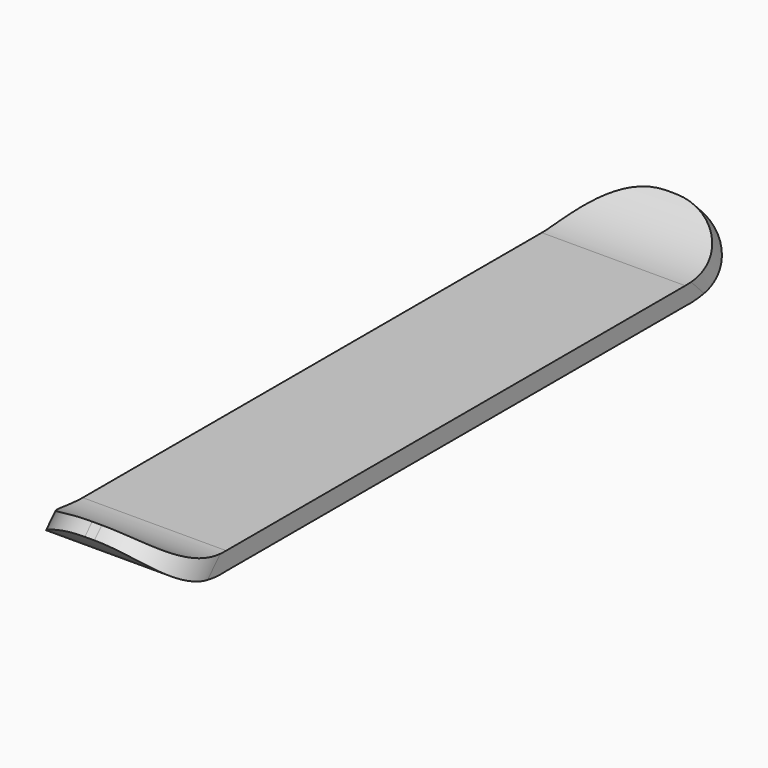
from build123d import *

# Parameters (mm, degrees)
F1_DEPTH    = 76.2
F2_T1_DEPTH = 369.824
F2_T3_DEPTH = 369.824


# Not quite as in the source:
# - a fillet or chamfer that OpenCascade refuses, or shapes differently, is made with other operations: its cross-section is extruded or revolved along the edge and cut away or added


with BuildPart() as f1:
    # F0 (on Right) → F1 (new body, symmetric)
    with BuildSketch(Plane.YZ):
        with BuildLine():
            Line((-304.8, 0), (0, 0))
            Line((0, 0), (304.8, 0))
            ThreePointArc((304.8, 0), (353.0430518596, 9.3618295777), (390.9983313803, 40.5777335736))
            Line((390.9983313803, 40.5777335736), (381.1075556217, 50.8))
            ThreePointArc((381.1075556217, 50.8), (346.1246462325, 27.304174222), (304.8, 19.05))
            Line((304.8, 19.05), (0, 19.05))
            Line((0, 19.05), (-304.8, 19.05))
            ThreePointArc((-304.8, 19.05), (-346.1246462325, 27.304174222), (-381.1075556217, 50.8))
            Line((-381.1075556217, 50.8), (-390.9983313803, 40.5777335736))
            ThreePointArc((-390.9983313803, 40.5777335736), (-353.0430518596, 9.3618295777), (-304.8, 0))
        make_face()
    extrude(amount=F1_DEPTH, both=True)

    # F2: fillet of radius 71.12 on 4 edges, made by hand

    # F2_s2 → F2_t1 (cut)
    with BuildSketch(Plane(origin=(0, -35.2534039099, -36.4349264406), x_dir=(1, 0, 0), z_dir=(0, -0.6953582507, -0.7186632752))):
        with BuildLine():
            ThreePointArc((5.08, 309.212203264), (55.369434278, 288.381637542), (76.2, 238.092203264))
            Line((76.2, 238.092203264), (76.2, 309.212203264))
            Line((76.2, 309.212203264), (5.08, 309.212203264))
        make_face()
        with BuildLine():
            ThreePointArc((-5.08, 309.212203264), (-55.369434278, 288.381637542), (-76.2, 238.092203264))
            Line((-76.2, 238.092203264), (-76.2, 309.212203264))
            Line((-76.2, 309.212203264), (-5.08, 309.212203264))
        make_face()
    extrude(amount=F2_T1_DEPTH, mode=Mode.SUBTRACT)

    # F2_s4 → F2_t3 (cut)
    with BuildSketch(Plane(origin=(0, 292.4135736338, -302.2138535277), x_dir=(1, 0, 0), z_dir=(0, -0.6953582507, 0.7186632752))):
        with BuildLine():
            ThreePointArc((5.08, 309.212203264), (55.369434278, 288.381637542), (76.2, 238.092203264))
            Line((76.2, 238.092203264), (76.2, 309.212203264))
            Line((76.2, 309.212203264), (5.08, 309.212203264))
        make_face()
        with BuildLine():
            ThreePointArc((-5.08, 309.212203264), (-55.369434278, 288.381637542), (-76.2, 238.092203264))
            Line((-76.2, 238.092203264), (-76.2, 309.212203264))
            Line((-76.2, 309.212203264), (-5.08, 309.212203264))
        make_face()
    extrude(amount=F2_T3_DEPTH, mode=Mode.SUBTRACT)


solid = f1.part
